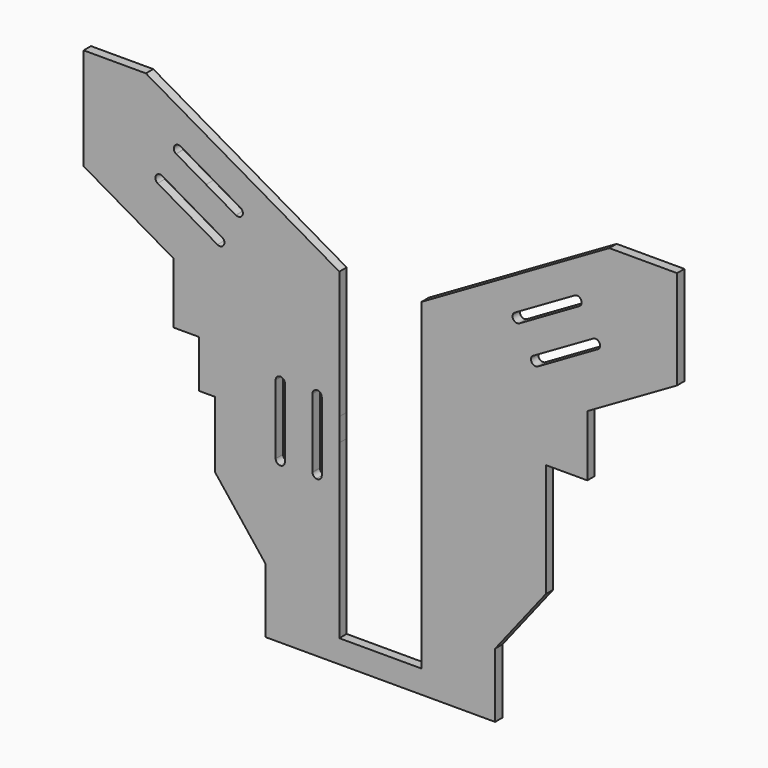
from build123d import *

# Parameters (mm, degrees)
F0_W     = 139
F0_H     = 20
F0_W_2   = 5
F0_H_2   = 350
F0_W_3   = 17.2517846753
F0_H_3   = 51.5162105877
F1_DEPTH = 10


# Not quite as in the source:
# - ends of sketch curves that miss each other by under 0.0002 mm in the source are joined


with BuildPart() as f1:
    # F0 (on Front) → F1 (new body)
    with BuildSketch(Plane.XZ):
        with BuildLine():
            Line((-52.4642963479, 111.8511321076), (-67.4642963479, 111.8511321076))
            Line((-67.4642963479, 111.8511321076), (-67.4642963479, 97.4173753779))
            Line((-67.4642963479, 97.4173753779), (-67.4642963479, -9.2363956308))
            ThreePointArc((-67.4642963479, -9.2363956308), (-63.3020069333, -10.2623815288), (-61.4642769098, -14.1353711486))
            ThreePointArc((-61.4642769098, -14.1353711486), (-61.4644203334, -14.1732421769), (-61.4648505957, -14.2111110326))
            Line((-61.4648505957, -14.2111110326), (-61.4659559185, -51.6353711486))
            Line((-61.4659559185, -51.6353711486), (-47.4642963479, -51.6353711486))
            Line((-47.4642963479, -51.6353711486), (-47.4642963479, 111.8511321076))
            Line((-47.4642963479, 111.8511321076), (-52.4642963479, 111.8511321076))
        make_face()
        Polygon((-67.4642963479, 97.4173753779), (-67.4642963479, 111.8511321076), (-52.4642963479, 111.8511321076), (-254.7302662373, 228.6294442711), (-264.7302662373, 211.3089361954), (-179.0455194088, 161.8388245486), align=None)
        with BuildLine():
            Line((-67.4642963479, -9.2363956308), (-67.4642963479, 97.4173753779))
            Line((-67.4642963479, 97.4173753779), (-179.0455194088, 161.8388245486))
            Line((-179.0455194088, 161.8388245486), (-182.0195368853, 156.6876751766))
            Line((-182.0195368853, 156.6876751766), (-149.6885534271, 138.0200999612))
            ThreePointArc((-149.6885534271, 138.0200999612), (-147.754915652, 136.1808734705), (-147.0427447391, 133.6090022218))
            ThreePointArc((-147.0427447391, 133.6090022218), (-149.4708734904, 129.3211731347), (-154.3969360511, 129.1979044824))
            ThreePointArc((-154.3969360511, 129.1979044824), (-154.5427447391, 129.2788752028), (-154.685771784, 129.3646638705))
            Line((-154.685771784, 129.3646638705), (-187.0173065595, 148.0312841764))
            Line((-187.0173065595, 148.0312841764), (-202.0308315575, 122.0270960791))
            Line((-202.0308315575, 122.0270960791), (-170.1659063917, 103.6023660524))
            ThreePointArc((-170.1659063917, 103.6023660524), (-169.5399428743, 103.2964942228), (-168.9625725467, 102.9065821737))
            ThreePointArc((-168.9625725467, 102.9065821737), (-167.5482558381, 101.1587780548), (-167.0427447391, 98.9679860704))
            ThreePointArc((-167.0427447391, 98.9679860704), (-169.5427447391, 94.6378590515), (-174.5427447391, 94.6378590515))
            Line((-174.5427447391, 94.6378590515), (-207.018697381, 113.3878590515))
            Line((-207.018697381, 113.3878590515), (-222.518697381, 86.5410715342))
            Line((-222.518697381, 86.5410715342), (-222.518697381, 66.1286172816))
            Line((-222.518697381, 66.1286172816), (-222.518697381, 46.1286172816))
            Line((-222.518697381, 46.1286172816), (-177.4642963479, 20.116446717))
            Line((-177.4642963479, 20.116446717), (-111.4642769098, -17.9886822721))
            Line((-111.4642769098, -17.9886822721), (-111.4642769098, -14.1353711486))
            ThreePointArc((-111.4642769098, -14.1353711486), (-106.4642769098, -9.1353711486), (-101.4642769098, -14.1353711486))
            Line((-101.4642769098, -14.1353711486), (-71.4642769098, -14.1353711486))
            ThreePointArc((-71.4642769098, -14.1353711486), (-71.4635814507, -14.0519798555), (-71.4614952667, -13.9686117605))
            ThreePointArc((-71.4614952667, -13.9686117605), (-70.283986672, -10.9089462954), (-67.4642963479, -9.2363956308))
        make_face()
        Polygon((-254.7302662373, 228.6294442711), (-52.4642963479, 111.8511321076), (-47.4642963479, 111.8511321076), (-42.4642963479, 111.8511321076), (-252.2302662373, 232.95957129), align=None)
        with BuildLine():
            Line((-182.0195368853, 156.6876751766), (-179.0455194088, 161.8388245486))
            Line((-179.0455194088, 161.8388245486), (-264.7302662373, 211.3089361954))
            Line((-264.7302662373, 211.3089361954), (-302.2302662373, 232.95957129))
            Line((-302.2302662373, 232.95957129), (-319.7805383214, 232.95957129))
            Line((-319.7805383214, 232.95957129), (-319.7805383214, 122.2827673304))
            Line((-319.7805383214, 122.2827673304), (-311.1202842835, 117.2827673304))
            Line((-311.1202842835, 117.2827673304), (-222.518697381, 66.1286172816))
            Line((-222.518697381, 66.1286172816), (-222.518697381, 86.5410715342))
            Line((-222.518697381, 86.5410715342), (-207.018697381, 113.3878590515))
            Line((-207.018697381, 113.3878590515), (-239.4946500229, 132.1378590515))
            ThreePointArc((-239.4946500229, 132.1378590515), (-241.3247770419, 138.9679860704), (-234.4946500229, 140.7981130893))
            Line((-234.4946500229, 140.7981130893), (-219.4946500229, 166.7788752029))
            ThreePointArc((-219.4946500229, 166.7788752029), (-219.5665212716, 166.8211731347), (-219.6376770678, 166.8646638705))
            ThreePointArc((-219.6376770678, 166.8646638705), (-221.6986741524, 169.4142582916), (-221.7372907101, 172.6924665608))
            ThreePointArc((-221.7372907101, 172.6924665608), (-218.7321520995, 175.7974013658), (-214.4293442023, 175.4007624721))
            Line((-214.4293442023, 175.4007624721), (-182.0195368853, 156.6876751766))
        make_face()
        Polygon((-42.4642963479, 111.8511321076), (-47.4642963479, 111.8511321076), (-47.4642963479, -51.6353711486), (-42.4642769098, -51.6353711486), (-42.4642963479, -26.6353711486), align=None)
        Polygon((-264.7302662373, 211.3089361954), (-254.7302662373, 228.6294442711), (-262.2302662373, 232.95957129), (-302.2302662373, 232.95957129), align=None)
        Polygon((-262.2302662373, 232.95957129), (-254.7302662373, 228.6294442711), (-252.2302662373, 232.95957129), align=None)
        Polygon((-42.4642769098, -51.6353711486), (-47.4642963479, -51.6353711486), (-47.4642963479, -238.1488678924), (-42.4642963479, -238.1488678924), align=None)
        with BuildLine():
            Line((-47.4642963479, -238.1488678924), (-47.4642963479, -51.6353711486))
            Line((-47.4642963479, -51.6353711486), (-61.4659559185, -51.6353711486))
            Line((-61.4659559185, -51.6353711486), (-61.4670585529, -88.9686117605))
            ThreePointArc((-61.4670585529, -88.9686117605), (-61.464972369, -89.0519798555), (-61.4642769098, -89.1353711486))
            ThreePointArc((-61.4642769098, -89.1353711486), (-63.3020069333, -93.0083607684), (-67.4642963479, -94.0343466663))
            Line((-67.4642963479, -94.0343466663), (-67.4642963479, -98.048845338))
            Line((-67.4642963479, -98.048845338), (-67.4642963479, -123.1488678924))
            Line((-67.4642963479, -123.1488678924), (-67.4642963479, -238.1488678924))
            Line((-67.4642963479, -238.1488678924), (-47.4642963479, -238.1488678924))
        make_face()
        with BuildLine():
            ThreePointArc((-71.4614952667, -14.3021305367), (-71.4635814507, -14.2187624417), (-71.4642769098, -14.1353711486))
            Line((-71.4642769098, -14.1353711486), (-101.4642762117, -14.1353711486))
            Line((-101.4642762117, -14.1353711486), (-101.4705038559, -23.758589835))
            Line((-101.4705038559, -23.758589835), (-71.4614952667, -41.0842990221))
            Line((-71.4614952667, -41.0842990221), (-71.4614952667, -14.3021305367))
        make_face()
        Polygon((-42.4642963479, -238.1488678924), (-47.4642963479, -238.1488678924), (-67.4642963479, -238.1488678924), (-67.4642963479, -243.1488678924), (71.5357036521, -243.1488678924), (71.5357036521, -238.1488678924), (51.5357036521, -238.1488678924), (46.5357036521, -238.1488678924), align=None)
        Polygon((-67.4642963479, -243.1488678924), (-67.4642963479, -238.1488678924), (-67.4642963479, -123.1488678924), (-177.4642963479, -123.1488678924), (-122.4642963479, -193.1488678924), (-67.4642963479, -263.1488678924), align=None)
        with BuildLine():
            Line((-71.4614952667, -88.9686117605), (-71.4614952667, -41.0842990221))
            Line((-71.4614952667, -41.0842990221), (-101.4705038559, -23.758589835))
            Line((-101.4705038559, -23.758589835), (-101.5123669409, -88.4435708452))
            ThreePointArc((-101.5123669409, -88.4435708452), (-101.4763139065, -88.7886362676), (-101.4642769098, -89.1353711486))
            ThreePointArc((-101.4642769098, -89.1353711486), (-101.4765393523, -89.4853340862), (-101.5132665329, -89.8335804636))
            ThreePointArc((-101.5132665329, -89.8335804636), (-106.8142398474, -94.1231087061), (-111.4642769098, -89.1353711486))
            Line((-111.4642769098, -89.1353711486), (-111.4642769098, -17.9886822721))
            Line((-111.4642769098, -17.9886822721), (-177.4642963479, 20.116446717))
            Line((-177.4642963479, 20.116446717), (-177.4642963479, 0))
            Line((-177.4642963479, 0), (-177.4642963479, -51.5162105877))
            Line((-177.4642963479, -51.5162105877), (-177.4642963479, -123.1488678924))
            Line((-177.4642963479, -123.1488678924), (-67.4642963479, -123.1488678924))
            Line((-67.4642963479, -123.1488678924), (-67.4642963479, -98.048845338))
            Line((-67.4642963479, -98.048845338), (-67.4642963479, -94.0343466663))
            ThreePointArc((-67.4642963479, -94.0343466663), (-70.283986672, -92.3617960018), (-71.4614952667, -89.3021305367))
            ThreePointArc((-71.4614952667, -89.3021305367), (-71.4642769098, -89.1353711486), (-71.4614952667, -88.9686117605))
        make_face()
        with BuildLine():
            Line((-202.0308315575, 122.0270960791), (-187.0173065595, 148.0312841764))
            Line((-187.0173065595, 148.0312841764), (-219.348841335, 166.6979044824))
            ThreePointArc((-219.348841335, 166.6979044824), (-219.4220833151, 166.7377818416), (-219.4946500229, 166.7788752029))
            Line((-219.4946500229, 166.7788752029), (-234.4946494994, 140.7981139961))
            Line((-234.4946494994, 140.7981139961), (-202.0308315575, 122.0270960791))
        make_face()
        with Locations((2.0357036521, -253.1488678924)):
            Rectangle(F0_W, F0_H)
        with Locations((49.0357036521, -63.1488678924)):
            Rectangle(F0_W_2, F0_H_2)
        Polygon((-122.4642963479, -263.1488678924), (-67.4642963479, -263.1488678924), (-122.4642963479, -193.1488678924), align=None)
        Polygon((71.5357036521, -238.1488678924), (71.5357036521, -243.1488678924), (71.5357036521, -263.1488678924), (126.5357036521, -193.1488678924), (181.5357036521, -123.1488678924), (71.5357036521, -123.1488678924), align=None)
        Polygon((51.5357036521, 111.8511321076), (51.5357036521, -238.1488678924), (71.5357036521, -238.1488678924), (71.5357036521, -123.1488678924), (71.5357036521, -43.3920828938), (71.5357036521, 97.4173753779), (71.5357036521, 111.8511321076), (56.5357036521, 111.8511321076), align=None)
        Polygon((250.3796616473, 229.5404961288), (46.5357036521, 111.8511321076), (51.5357036521, 111.8511321076), (56.5357036521, 111.8511321076), (252.8796616473, 225.2103691099), align=None)
        Polygon((-177.4642963479, 0), (-177.4642963479, 20.116446717), (-222.518697381, 46.1286172816), (-222.518697381, 0), (-194.7160810232, 0), align=None)
        with Locations((-186.0901886856, -25.7581052938)):
            Rectangle(F0_W_3, F0_H_3)
        Polygon((126.5357036521, -193.1488678924), (71.5357036521, -263.1488678924), (126.5357036521, -263.1488678924), align=None)
        Polygon((260.3796616473, 229.5404961288), (250.3796616473, 229.5404961288), (252.8796616473, 225.2103691099), align=None)
        Polygon((71.5357036521, -43.3920828938), (71.5357036521, -123.1488678924), (181.5357036521, -123.1488678924), (181.5357036521, 0), (181.5357036521, 20.116446717), align=None)
        Polygon((252.8796616473, 225.2103691099), (56.5357036521, 111.8511321076), (71.5357036521, 111.8511321076), (71.5357036521, 97.4173753779), (177.45381959, 158.5692281267), (262.8796616473, 207.8898610342), align=None)
        Polygon((260.3796616473, 229.5404961288), (252.8796616473, 225.2103691099), (262.8796616473, 207.8898610342), (300.3796616473, 229.5404961288), align=None)
        Polygon((71.5357036521, 97.4173753779), (71.5357036521, -43.3920828938), (181.5357036521, 20.116446717), (226.5901036521, 46.1286166852), (226.5901036521, 66.1286166852), (315.1916915876, 117.2827673304), (262.8796616473, 207.8898610342), (177.45381959, 158.5692281267), align=None)
        with BuildLine():
            ThreePointArc((172.950565815, 91.3690924644), (166.120438796, 93.1992194834), (167.950565815, 100.0293465023))
            Line((167.950565815, 100.0293465023), (232.3273994773, 137.141799162))
            ThreePointArc((232.3273994773, 137.141799162), (232.9052740107, 137.5309635551), (233.5316329143, 137.8360249017))
            ThreePointArc((233.5316329143, 137.8360249017), (238.1994166719, 137.3437454468), (240.4024710988, 133.1992194834))
            ThreePointArc((240.4024710988, 133.1992194834), (239.7325981177, 130.6992194834), (237.9024710988, 128.8690924644))
            Line((237.9024710988, 128.8690924644), (172.950565815, 91.3690924644))
        make_face(mode=Mode.SUBTRACT)
        with BuildLine():
            Line((148.0164453216, 134.7077357691), (180.4273579612, 153.4189085895))
            Line((180.4273579612, 153.4189085895), (212.7594440539, 172.084573986))
            ThreePointArc((212.7594440539, 172.084573986), (217.829904391, 172.2114560149), (220.4024710988, 167.8402356347))
            ThreePointArc((220.4024710988, 167.8402356347), (219.773691479, 165.4128023426), (218.0454981437, 163.5958972835))
            ThreePointArc((218.0454981437, 163.5958972835), (217.9024710988, 163.5101086158), (217.7566624108, 163.4291378954))
            Line((217.7566624108, 163.4291378954), (153.0935928598, 126.0958972835))
            ThreePointArc((153.0935928598, 126.0958972835), (153.0224370637, 126.0524065477), (152.950565815, 126.0101086158))
            ThreePointArc((152.950565815, 126.0101086158), (152.8779991071, 125.9690152546), (152.804757127, 125.9291378954))
            ThreePointArc((152.804757127, 125.9291378954), (146.061084943, 127.945980495), (148.0164453216, 134.7077357691))
        make_face(mode=Mode.SUBTRACT)
        Polygon((300.3796616473, 229.5404961288), (262.8796616473, 207.8898610342), (315.1916915876, 117.2827673304), (323.8519456255, 122.2827673304), (323.8519456255, 229.5404961288), align=None)
        Polygon((181.5357036521, 20.116446717), (181.5357036521, 0), (226.5901036521, 0), (226.5901036521, 46.1286166852), align=None)
    extrude(amount=F1_DEPTH)


solid = f1.part
